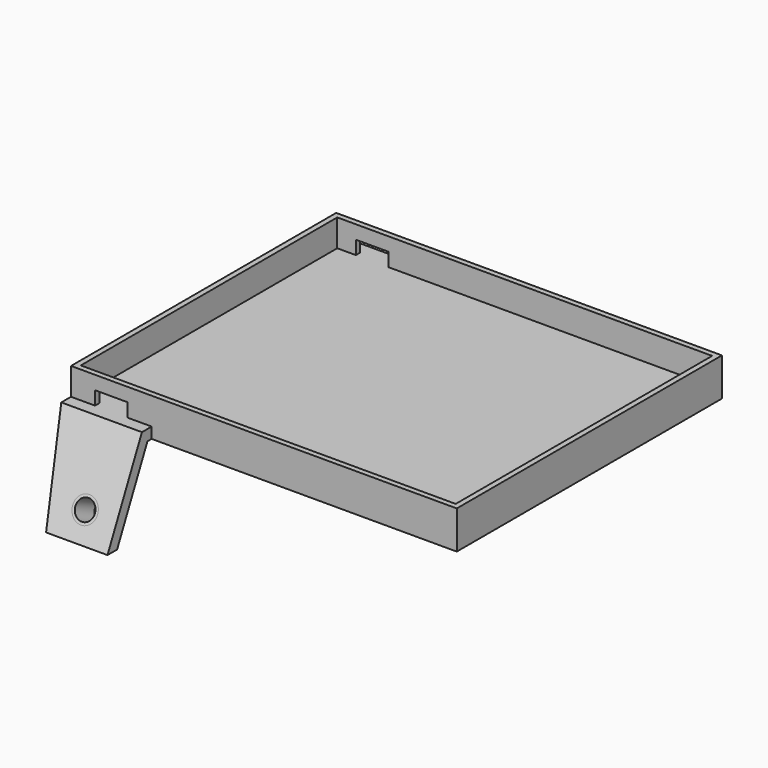
from build123d import *

# Parameters (mm, degrees)
F1_DEPTH      = 31.75
F2_R          = 0.127
F3_DEPTH      = 56.2093301913
F3_DEPTH_BACK = 56.2093301913
F4_W          = 90.17
F4_H          = 77.47
F5_DEPTH      = 2.54
F6_W          = 90.17
F6_H          = 77.47
F6_W_2        = 87.63
F6_H_2        = 74.93
F7_DEPTH      = 6.35
F11_W         = 7.62
F11_H         = 3.175
F12_DEPTH     = 79.756
F14_R         = 2.921
F14_R_2       = 2.286
F15_DEPTH     = 6.35
F15_FACE_R    = 2.286
F16_DEPTH     = 12.9286
F17_R         = 2.070357412
F18_DEPTH     = 25.4
F20_R         = 2.286
F21_DEPTH     = 25.4


# Not quite as in the source:
# - a pattern or mirror of a feature is missing from the dataset's text; its kind, count and spacing are read off the source's solid


with BuildPart() as f1:
    # F0 (on Right) → F1 (new body)
    with BuildSketch(Plane.YZ):
        Polygon((-53.9136660383, -18.1264164896), (-39.9723188616, 11.2473889307), (39.9723188616, 11.2473889307), (53.9136660383, -18.1264164896), (56.2083301913, -17.0373267665), (41.5783543673, 13.7873889307), (-41.5783543673, 13.7873889307), (-56.2083301913, -17.0373267665), align=None)
    extrude(amount=F1_DEPTH)

    # F2 (on Front) → F3 (cut, two sides)
    with BuildSketch(Plane.XZ) as f3_sk:
        Polygon((12.8995720297, 13.7873889307), (0, 13.7873889307), (0, -18.1264164896), (19.6673367172, -18.1264164896), (35.7595719397, -19.0736036748), (35.7595719397, -7.4199110855), (17.3968738801, -7.4199110855), align=None)
        with Locations((24.329572916, -1.6249689179)):
            Circle(F2_R)
    extrude(amount=-F3_DEPTH, mode=Mode.SUBTRACT)
    extrude(f3_sk.sketch, amount=F3_DEPTH_BACK, mode=Mode.SUBTRACT)

    # F4 (on face) → F5 (join, through all)
    with BuildSketch(Plane(origin=(0, 0, 11.2473889307), x_dir=(1, 0, 0), z_dir=(0, 0, -1))):
        with Locations((57.9845720297, 0)):
            Rectangle(F4_W, F4_H)
    extrude(amount=-F5_DEPTH)

    # F6 (on face) → F7 (join)
    with BuildSketch(Plane.XY.offset(13.7873889307)):
        with Locations((57.9845720297, 0)):
            Rectangle(F6_W, F6_H)
        with Locations((57.9845720297, 0)):
            Rectangle(F6_W_2, F6_H_2, mode=Mode.SUBTRACT)
    extrude(amount=F7_DEPTH)

    # F11 (on face) → F12 (cut)
    with BuildSketch(Plane(origin=(0, 38.735, 0), x_dir=(-1, 0, 0), z_dir=(0, 1, 0))):
        with Locations((-22.3247860149, 15.3748889307)):
            Rectangle(F11_W, F11_H)
    extrude(amount=-F12_DEPTH, mode=Mode.SUBTRACT)

    # F14 (on face) → F15 (join)
    with BuildSketch(Plane(origin=(0, 39.2749300586, 18.6406026544), x_dir=(-1, 0, 0), z_dir=(0, 0.9034110839, 0.4287754815))):
        with Locations((-24.329572916, -22.4322813106)):
            Circle(F14_R)
        with Locations((-24.329572916, -22.4322813106)):
            Circle(F14_R_2, mode=Mode.SUBTRACT)
    f15 = extrude(amount=-F15_DEPTH)

    # F15_copies: F15 across plane
    add(f15.mirror(Plane(origin=(0, 0, 0), x_dir=(0, 0, -1), z_dir=(0, -1, 0))))

    # F14 (on face) + F15_face (on face) → F16 (cut)
    with BuildSketch(Plane(origin=(0, 39.2749300586, 18.6406026544), x_dir=(-1, 0, 0), z_dir=(0, 0.9034110839, 0.4287754815))):
        with Locations((-24.329572916, -22.4322813106)):
            Circle(F14_R)
        with Locations((-24.329572916, -22.4322813106)):
            Circle(F14_R_2, mode=Mode.SUBTRACT)
    with BuildSketch(Plane(origin=(24.329572916, 46.6004501275, -2.7177921697), x_dir=(1, 0, 0), z_dir=(0, -0.9034110839, -0.4287754815))):
        with Locations((0, 0.004132702)):
            Circle(F15_FACE_R)
        with BuildLine():
            add(Edge.make_bspline(
                [(0.127, 1.2096633209), (0.127, 0.9661745521), (-0.0635, 1.0879189365), (-0.254, 1.2096633209), (-0.0635, 1.3314077053), (0.127, 1.4531520897), (0.127, 1.2096633209)],
                knots=[1.5707963268, 1.5707963268, 1.5707963268, 3.6651914292, 3.6651914292, 5.7595865316, 5.7595865316, 7.853981634, 7.853981634, 7.853981634], degree=2, weights=[1, 0.5, 1, 0.5, 1, 0.5, 1]))
        make_face(mode=Mode.SUBTRACT)
    extrude(amount=F16_DEPTH, dir=(0, 0.9034110839, 0.4287754815), mode=Mode.SUBTRACT)

    # F17 (on face) → F18 (cut)
    with BuildSketch(Plane(origin=(0, 33.5382696761, 15.9178783467), x_dir=(1, 0, 0), z_dir=(0, -0.9034110839, -0.4287754815))):
        with Locations((24.329572916, -22.4322813106)):
            Circle(F17_R)
    extrude(amount=-F18_DEPTH, mode=Mode.SUBTRACT)

    # F20 (on face) → F21 (cut)
    with BuildSketch(Plane(origin=(0, -36.9802659056, 17.5515129313), x_dir=(-1, 0, 0), z_dir=(0, 0.9034110839, -0.4287754815))):
        with Locations((-24.329572916, -22.4322813106)):
            Circle(F20_R)
    extrude(amount=-F21_DEPTH, mode=Mode.SUBTRACT)


solid = f1.part
